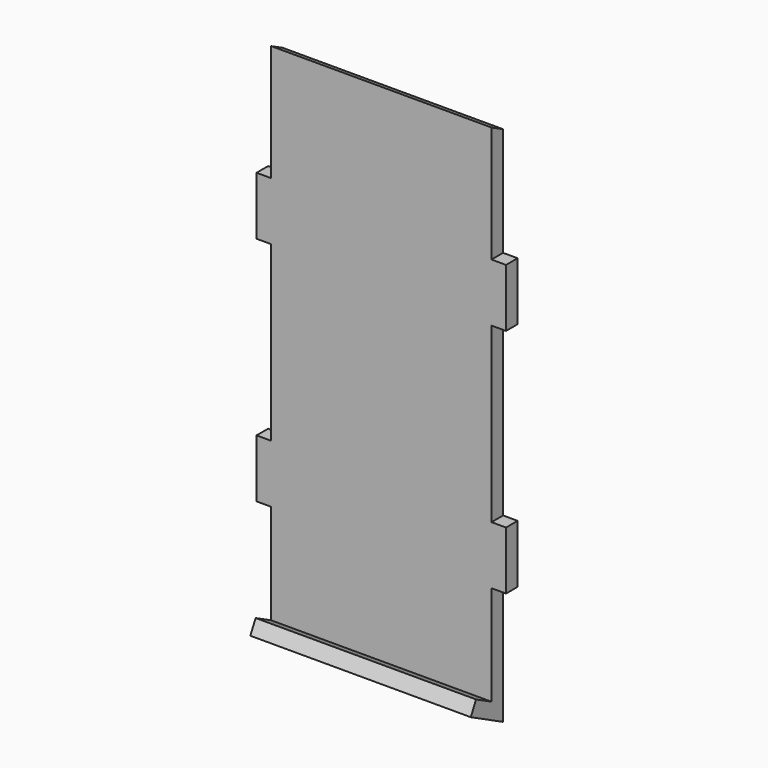
from build123d import *

# Parameters (mm, degrees)
F1_DEPTH = 3.175
F3_DEPTH = 43.942
F5_DEPTH = 76.2
F6_DEPTH = 48.1697538


# Not quite as in the source:
# - a feature names something its author has since deleted; it is built from what else it names


with BuildPart() as f1:
    # F0 (on Front) → F1 (new body)
    with BuildSketch(Plane.XZ):
        Polygon((-34.9639124011, -57.0107064), (9.4471751978, -57.0107064), (13.2058413989, -57.0107064), (13.2058413989, -31.6107064), (16.3808413989, -31.6107064), (16.3808413989, -18.9107064), (13.2058413989, -18.9107064), (13.2058413989, 18.9107064), (16.3808413989, 18.9107064), (16.3808413989, 31.6107064), (13.2058413989, 31.6107064), (13.2058413989, 57.0107064), (-34.9639124011, 57.0107064), (-34.9639124011, 31.6107064), (-38.1389124011, 31.6107064), (-38.1389124011, 18.9107064), (-34.9639124011, 18.9107064), (-34.9639124011, -18.9107064), (-38.1389124011, -18.9107064), (-38.1389124011, -31.6107064), (-34.9639124011, -31.6107064), align=None)
    extrude(amount=F1_DEPTH)

    # F2 (on face) → F3 (join)
    with BuildSketch(Plane(origin=(-34.9639124011, 0, 0), x_dir=(0, -1, 0), z_dir=(-1, 0, 0))):
        Polygon((0, -58.6279720227), (3.175, -57.0107064), (8.8332357394, -54.1285425744), (7.3921538265, -51.2994247047), (0, -55.0648030547), align=None)
    extrude(amount=-F3_DEPTH)

    # F4 (on face) → F5 (cut)
    with BuildSketch(Plane(origin=(-34.9639124011, 0, 0), x_dir=(0, -1, 0), z_dir=(-1, 0, 0))):
        Polygon((0, 55.3934407773), (3.175, 57.0107064), (0, 57.0107064), align=None)
    extrude(amount=-F5_DEPTH, mode=Mode.SUBTRACT)

    # F2 (on face) → F6 (join)
    with BuildSketch(Plane(origin=(-34.9639124011, 0, 0), x_dir=(0, -1, 0), z_dir=(-1, 0, 0))):
        Polygon((0, -58.6279720227), (3.175, -57.0107064), (8.8332357394, -54.1285425744), (7.3921538265, -51.2994247047), (0, -55.0648030547), align=None)
    extrude(amount=-F6_DEPTH)


solid = f1.part
